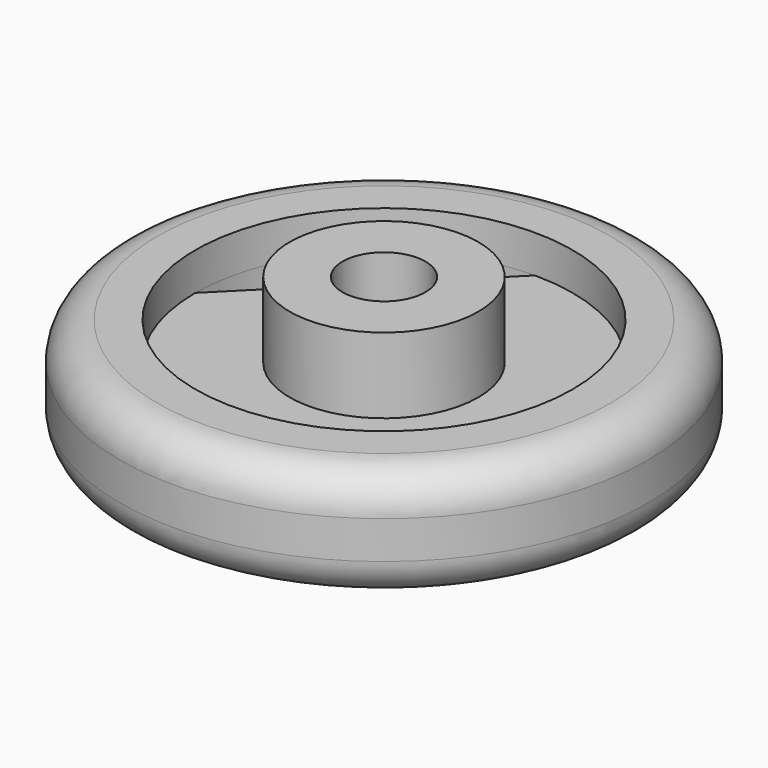
from build123d import *

# Parameters (mm, degrees)
F0_R          = 7
F0_R_2        = 5
F1_DEPTH      = 3
F2_START      = 1
F0_R_3        = 2.5
F2_DEPTH      = 1
F3_DEPTH      = 4
F3_DEPTH_BACK = 1
F5_D          = 2.2
F6_R          = 1
F8_DEPTH      = 3


with BuildPart() as f1:
    # F0 (on Top) → F1 (new body)
    with BuildSketch(Plane.XY):
        Circle(F0_R)
        Circle(F0_R_2, mode=Mode.SUBTRACT)
    extrude(amount=F1_DEPTH)

    # F0 (on Top) → F2 (join)
    with BuildSketch(Plane.XY.offset(F2_START)):
        Circle(F0_R_2)
        Circle(F0_R_3, mode=Mode.SUBTRACT)
    extrude(amount=F2_DEPTH)

    # F0 (on Top) → F3 (join, two sides)
    with BuildSketch(Plane.XY) as f3_sk:
        Circle(F0_R_3)
    extrude(amount=F3_DEPTH)
    extrude(f3_sk.sketch, amount=-F3_DEPTH_BACK)

    # F5 (through all)
    with Locations(Plane.XY.offset(4)):
        with Locations((0, 0)):
            Hole(F5_D / 2)

    # F6
    f6_edges = [f1.edges().sort_by_distance(p)[0] for p in [
        (-7, 0, 3),
        (-7, 0, 0),
    ]]
    fillet(f6_edges, radius=F6_R)

    # F7 (on face) → F8 (cut)
    with BuildSketch(Plane.XY.offset(2)):
        with BuildLine():
            Line((-5, 0), (0, 5))
            ThreePointArc((0, 5), (-3.535534, 3.535534), (-5, 0))
        make_face()
        with BuildLine():
            ThreePointArc((0, -5), (3.535534, -3.535534), (5, 0))
            Line((5, 0), (0, -5))
        make_face()
    extrude(amount=-F8_DEPTH, mode=Mode.SUBTRACT)


solid = f1.part
